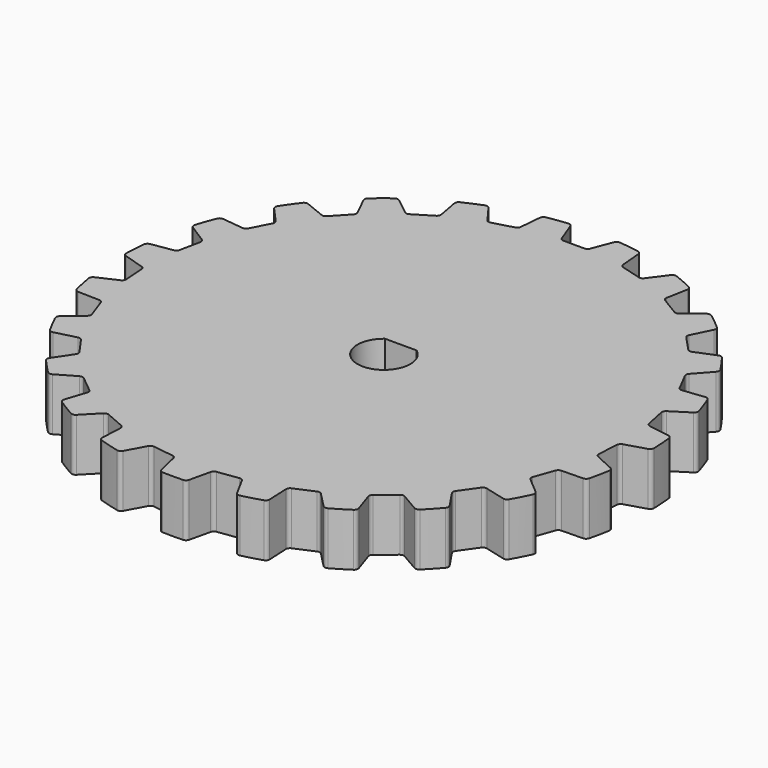
from build123d import *

# Parameters (mm, degrees)
F0_R      = 10
F1_DEPTH  = 2
F3_DEPTH  = 25
F4_COUNT  = 23
F5_R      = 0.15
F6_R      = 0.15
F7_R      = 0.15
F8_R      = 0.15
F10_DEPTH = 25


with BuildPart() as f1:
    # F0 (on Top) → F1 (new body)
    with BuildSketch(Plane.XY):
        Circle(F0_R)
    extrude(amount=F1_DEPTH)

    # F2 (on face) → F3 (cut)
    with BuildSketch(Plane.XY.offset(2)):
        with BuildLine():
            Line((0, 10), (0, 9))
            Line((0, 9), (0.5, 9))
            Line((0.5, 9), (0.8657328431, 9.9624548503))
            ThreePointArc((0.8657328431, 9.9624548503), (0.4332732954, 9.9906093033), (0, 10))
        make_face()
        with BuildLine():
            Line((-0.5, 9), (0, 9))
            Line((0, 9), (0, 10))
            ThreePointArc((0, 10), (-0.4332732954, 9.9906093033), (-0.8657328431, 9.9624548503))
            Line((-0.8657328431, 9.9624548503), (-0.5, 9))
        make_face()
    f3 = extrude(amount=-F3_DEPTH, mode=Mode.SUBTRACT)

    # F4: F3 ×23 about axis
    f4_axis = Axis((0, 0, 0), (0, 0, -1))
    for i in range(1, F4_COUNT):
        add(f3.rotate(f4_axis, i * 360 / F4_COUNT), mode=Mode.SUBTRACT)

    # F5
    f5_edges = [f1.edges().sort_by_distance(p)[0] for p in [
        (0.5, 9, 1),
        (-0.5, 9, 1),
        (0.865733, 9.962455, 1),
        (-0.865733, 9.962455, 1),
    ]]
    fillet(f5_edges, radius=F5_R)

    # F6
    f6_edges = [f1.edges().sort_by_distance(p)[0] for p in [
        (-1.854209, 9.826592, 1),
        (-1.946712, 8.801154, 1),
        (-2.90963, 8.531357, 1),
        (-3.521467, 9.359448, 1),
        (-4.436633, 8.961936, 1),
        (-4.249046, 7.949567, 1),
        (-5.103465, 7.429983, 1),
        (-5.916031, 8.062294, 1),
        (-6.690012, 7.432614, 1),
        (-6.236247, 6.508396, 1),
        (-6.9188, 5.77756, 1),
        (-7.871829, 6.167196, 1),
        (-8.447223, 5.352049, 1),
        (-7.760934, 4.584528, 1),
        (-8.220999, 3.696643, 1),
        (-9.24381, 3.814706, 1),
    ]]
    fillet(f6_edges, radius=F6_R)

    # F7
    f7_edges = [f1.edges().sort_by_distance(p)[0] for p in [
        (1.854209, 9.826592, 1),
        (1.946712, 8.801154, 1),
        (2.90963, 8.531357, 1),
        (3.521467, 9.359448, 1),
        (4.436633, 8.961936, 1),
        (5.103465, 7.429983, 1),
        (4.249046, 7.949567, 1),
        (5.916031, 8.062294, 1),
        (6.690012, 7.432614, 1),
        (6.236247, 6.508396, 1),
        (6.9188, 5.77756, 1),
        (7.871829, 6.167196, 1),
        (8.447223, 5.352049, 1),
        (7.760934, 4.584528, 1),
        (8.220999, 3.696643, 1),
        (9.24381, 3.814706, 1),
        (9.577942, 2.874547, 1),
        (8.710029, 2.320646, 1),
        (8.913485, 1.341562, 1),
        (9.93022, 1.179296, 1),
        (9.99831, 0.183853, 1),
        (9.01314, -0.115347, 1),
        (8.944898, -1.113016, 1),
        (9.88015, -1.543577, 1),
        (9.677148, -2.520477, 1),
        (8.647788, -2.542786, 1),
    ]]
    fillet(f7_edges, radius=F7_R)

    # F8
    f8_edges = [f1.edges().sort_by_distance(p)[0] for p in [
        (8.312908, -3.485047, 1),
        (9.097316, -4.151969, 1),
        (8.638277, -5.037874, 1),
        (7.641069, -4.781638, 1),
        (7.064389, -5.598608, 1),
        (7.639775, -6.452429, 1),
        (6.958744, -7.181635, 1),
        (6.067647, -6.665858, 1),
        (5.291936, -7.296946, 1),
        (5.615626, -8.274342, 1),
        (4.763113, -8.792767, 1),
        (4.044215, -8.055701, 1),
        (3.127004, -8.454102, 1),
        (3.174993, -9.482585, 1),
        (2.214223, -9.75178, 1),
        (1.720843, -8.84809, 1),
        (0.498885, -9.987548, 1),
        (0.730157, -8.984257, 1),
        (-0.498885, -9.987548, 1),
        (-0.730157, -8.984257, 1),
        (-1.720843, -8.84809, 1),
        (-2.214223, -9.75178, 1),
        (-3.174993, -9.482585, 1),
        (-3.127004, -8.454102, 1),
        (-4.763113, -8.792767, 1),
        (-5.615626, -8.274342, 1),
        (-5.291936, -7.296946, 1),
        (-6.067647, -6.665858, 1),
        (-6.958744, -7.181635, 1),
        (-7.639775, -6.452429, 1),
        (-7.641069, -4.781638, 1),
        (-8.638277, -5.037874, 1),
        (-8.647788, -2.542786, 1),
        (-9.677148, -2.520477, 1),
        (-9.01314, -0.115347, 1),
        (-9.99831, 0.183853, 1),
        (-9.93022, 1.179296, 1),
        (-9.097316, -4.151969, 1),
        (-9.88015, -1.543577, 1),
        (-7.064389, -5.598608, 1),
        (-4.044215, -8.055701, 1),
        (-8.312908, -3.485047, 1),
        (-8.944898, -1.113016, 1),
        (-8.913485, 1.341562, 1),
        (-8.710029, 2.320646, 1),
        (-9.577942, 2.874547, 1),
    ]]
    fillet(f8_edges, radius=F8_R)

    # F9 (on face) → F10 (cut)
    with BuildSketch(Plane.XY.offset(2)):
        with BuildLine():
            ThreePointArc((-0.6, 0.8), (-0.4472135955, -0.894427191), (1, 0))
            ThreePointArc((1, 0), (0.894427191, 0.4472135955), (0.6, 0.8))
            Line((0.6, 0.8), (0, 0.8))
            Line((0, 0.8), (-0.6, 0.8))
        make_face()
    extrude(amount=-F10_DEPTH, mode=Mode.SUBTRACT)


solid = f1.part
